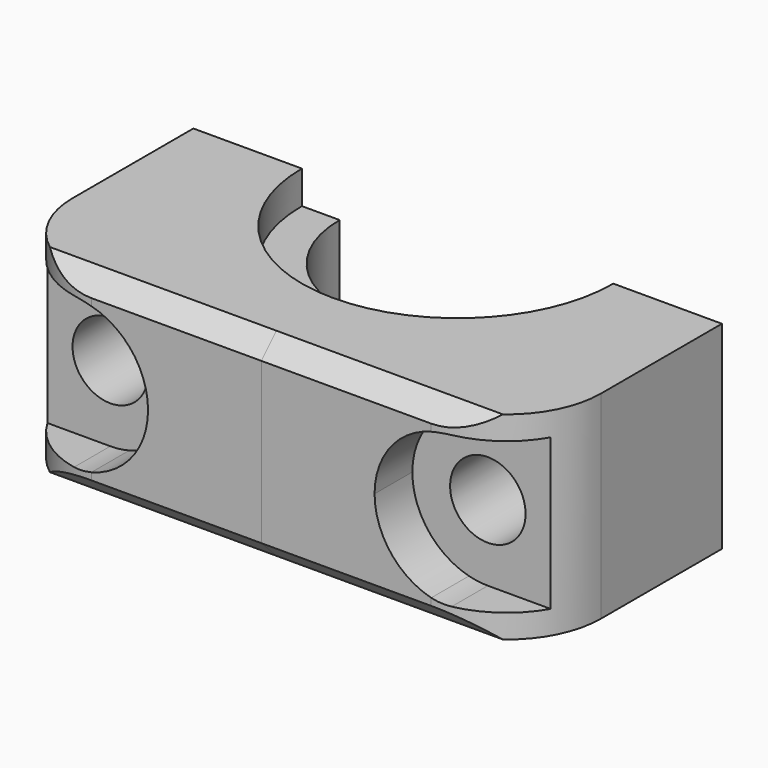
from build123d import *

# Parameters (mm, degrees)
F0_R        = 2
F0_W        = 6.25
F0_H        = 5.75
F1_DEPTH    = 13
F3_DEPTH    = 25
F4_T1_DEPTH = 35.5
F6_DEPTH    = 2.5
F7_T1_DEPTH = 15.9435440675


# Not quite as in the source:
# - a fillet or chamfer that OpenCascade refuses, or shapes differently, is made with other operations: its cross-section is extruded or revolved along the edge and cut away or added


with BuildPart() as f1:
    # F0 (on Front) → F1 (new body)
    with BuildSketch(Plane.XZ):
        Polygon((-8.25, 3.5), (-8.25, 5.25), (-14, 5.25), (-14, -5.25), (-8.25, -5.25), (-8.25, -2.25), (-6.25, -2.25), (-6.25, 3.5), align=None)
        with Locations((-10, 0)):
            Circle(F0_R, mode=Mode.SUBTRACT)
        with Locations((-10, 0)):
            Circle(F0_R)
        Polygon((0, 3.5), (0, 5.25), (-8.25, 5.25), (-8.25, 3.5), (-6.25, 3.5), align=None)
        with Locations((-3.125, 0.625)):
            Rectangle(F0_W, F0_H)
        Polygon((0, -5.25), (0, -2.25), (-6.25, -2.25), (-8.25, -2.25), (-8.25, -5.25), align=None)
    extrude(amount=F1_DEPTH)

    # F0 (on Front) → F2 (revolve, cut)
    with BuildSketch(Plane.XZ):
        Polygon((0, 3.5), (0, 5.25), (-8.25, 5.25), (-8.25, 3.5), (-6.25, 3.5), align=None)
        with Locations((-3.125, 0.625)):
            Rectangle(F0_W, F0_H)
        Polygon((0, -5.25), (0, -2.25), (-6.25, -2.25), (-8.25, -2.25), (-8.25, -5.25), align=None)
    revolve(axis=Axis((0, 0, 0), (0, 0, -1)), mode=Mode.SUBTRACT)

    # F0 (on Front) → F3 (cut)
    with BuildSketch(Plane.XZ):
        with Locations((-10, 0)):
            Circle(F0_R)
    extrude(amount=F3_DEPTH, mode=Mode.SUBTRACT)

    # F4: fillet of radius 5 on 1 edges, made by hand

    # F4_s2 → F4_t1 (cut)
    with BuildSketch(Plane.XY.offset(-17.75)):
        with BuildLine():
            ThreePointArc((-14, -8), (-12.5355339059, -11.5355339059), (-9, -13))
            Line((-9, -13), (-14, -13))
            Line((-14, -13), (-14, -8))
        make_face()
    extrude(amount=F4_T1_DEPTH, mode=Mode.SUBTRACT)

    # F5 (on face) → F6 (cut)
    with BuildSketch(Plane.XZ.offset(13)):
        with BuildLine():
            Line((-17.9225690663, -4), (-10, -4))
            ThreePointArc((-10, -4), (-12.8284271247, -2.8284271247), (-14, 0))
            Line((-14, 0), (-17.9225690663, 0))
            Line((-17.9225690663, 0), (-17.9225690663, -4))
        make_face()
        with BuildLine():
            ThreePointArc((-14, 0), (-12.8284271247, 2.8284271247), (-10, 4))
            Line((-10, 4), (-17.9225690663, 4))
            Line((-17.9225690663, 4), (-17.9225690663, 0))
            Line((-17.9225690663, 0), (-14, 0))
        make_face()
        with BuildLine():
            Line((-10, 0), (-10, 4))
            ThreePointArc((-10, 4), (-12.8284271247, 2.8284271247), (-14, 0))
            Line((-14, 0), (-10, 0))
        make_face()
        with BuildLine():
            ThreePointArc((-9, -3.8729833462), (-6.8377223398, -2.4494897428), (-6, 0))
            ThreePointArc((-6, 0), (-6.8377223398, 2.4494897428), (-9, 3.8729833462))
            Line((-9, 3.8729833462), (-9, 1.7320508076))
            ThreePointArc((-9, 1.7320508076), (-8.2679491924, 1), (-8, 0))
            ThreePointArc((-8, 0), (-8.2679491924, -1), (-9, -1.7320508076))
            Line((-9, -1.7320508076), (-9, -3.8729833462))
        make_face()
        with BuildLine():
            Line((-9, 1.7320508076), (-9, 3.8729833462))
            ThreePointArc((-9, 3.8729833462), (-9.4959828301, 3.9681187851), (-10, 4))
            Line((-10, 4), (-10, 0))
            Line((-10, 0), (-10, -4))
            ThreePointArc((-10, -4), (-9.4959828301, -3.9681187851), (-9, -3.8729833462))
            Line((-9, -3.8729833462), (-9, -1.7320508076))
            ThreePointArc((-9, -1.7320508076), (-8.2679491924, -1), (-8, 0))
            ThreePointArc((-8, 0), (-8.2679491924, 1), (-9, 1.7320508076))
        make_face()
        with BuildLine():
            ThreePointArc((-14, 0), (-12.8284271247, -2.8284271247), (-10, -4))
            Line((-10, -4), (-10, 0))
            Line((-10, 0), (-14, 0))
        make_face()
    extrude(amount=-F6_DEPTH, mode=Mode.SUBTRACT)

    # F7: chamfer of 1 on 2 edges, made by hand

    # F7_s2 → F7_t1 (cut)
    with BuildSketch(Plane.YZ.offset(-13.3718610795)):
        Polygon((-12, -5.25), (-13, -4.25), (-13, -5.25), align=None)
        Polygon((-12, 5.25), (-13, 4.25), (-13, 5.25), align=None)
    extrude(amount=F7_T1_DEPTH, mode=Mode.SUBTRACT)

    # F8: F1 across face


with BuildPart() as f1_1:
    add(f1.part)
    add(f1.part.mirror(Plane(origin=(0, -9.948326432, 0.119047619), x_dir=(0, 1, 0), z_dir=(1, 0, 0))))


solid = f1_1.part
